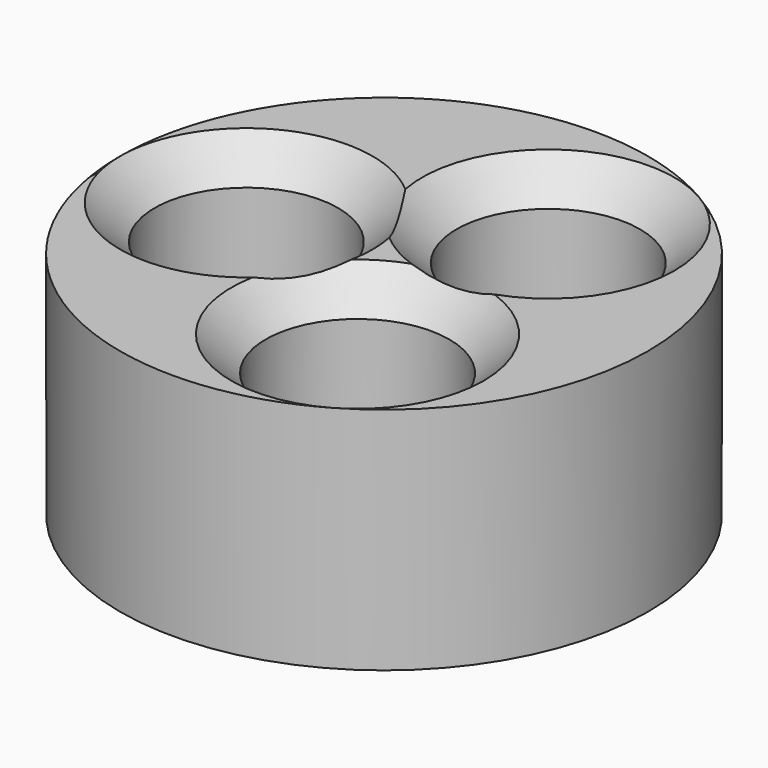
from build123d import *

# Parameters (mm, degrees)
F0_R     = 14.605
F0_R_2   = 5.08
F1_DEPTH = 12.7
F2_SIZE  = 1.90499


# Not quite as in the source:
# - a fillet or chamfer that OpenCascade refuses, or shapes differently, is made with other operations: its cross-section is extruded or revolved along the edge and cut away or added
# - a fillet or chamfer is up to 0.001 mm smaller than in the source, because OpenCascade refuses the exact size


with BuildPart() as f1:
    # F0 (on Top) → F1 (new body)
    with BuildSketch(Plane.XY):
        Circle(F0_R)
        with Locations((-7.62, 0)):
            Circle(F0_R_2, mode=Mode.SUBTRACT)
        with Locations((3.81, -6.5991135768)):
            Circle(F0_R_2, mode=Mode.SUBTRACT)
        with Locations((3.81, 6.5991135768)):
            Circle(F0_R_2, mode=Mode.SUBTRACT)
    extrude(amount=F1_DEPTH)

    # F2 (size 1.905 in the source; OpenCascade refuses exactly that, so slightly less here)
    f2_edges = [f1.edges().sort_by_distance(p)[0] for p in [
        (-12.7, 0, 12.7),
    ]]
    chamfer(f2_edges, length=F2_SIZE)

    # F3: chamfer of 1.905 on 1 edges, made by hand

    # F3_s1 → F3_t2 (revolve, cut)
    with BuildSketch(Plane.XZ.offset(-6.5991135768)):
        Polygon((10.795, 12.7), (8.89, 10.795), (8.89, 12.7), align=None)
    revolve(axis=Axis((3.81, 6.5991135768, 12.7), (0, 0, 1)), mode=Mode.SUBTRACT)

    # F4: chamfer of 1.905 on 1 edges, made by hand

    # F4_s1 → F4_t2 (revolve, cut)
    with BuildSketch(Plane.XZ.offset(6.5991135768)):
        Polygon((10.795, 12.7), (8.89, 10.795), (8.89, 12.7), align=None)
    revolve(axis=Axis((3.81, -6.5991135768, 12.7), (0, 0, 1)), mode=Mode.SUBTRACT)


solid = f1.part
